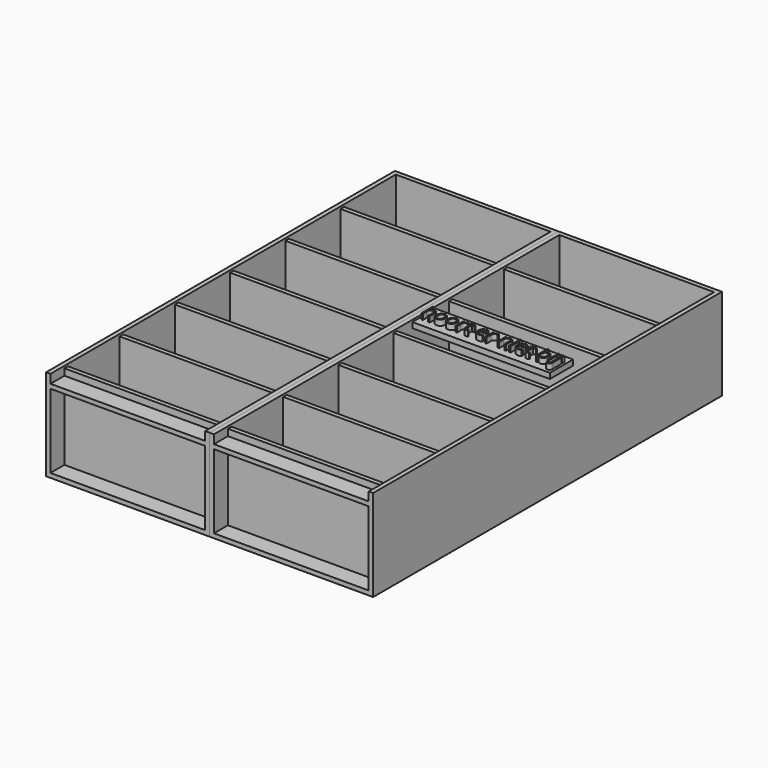
from build123d import *

# Parameters (mm, degrees)
F1_DEPTH      = 400
F3_W          = 630.7227015495
F3_H          = 132.8808516264
F4_DEPTH      = 25
F0_W          = 710
F0_H          = 20
F5_DEPTH      = 390
F6_W          = 710
F6_H          = 20
F7_DEPTH      = 80
F9_DEPTH      = 2000
F11_TEXT_SIZE = 85.9931443582
F12_DEPTH     = 25


# Not quite as in the source:
# - Text() gives the source's letters only with a copy of the font that has no kerning and outlines rounded to 1/6400 em; it was checked with that copy


with BuildPart() as f1:
    # F0 (on Top) → F1 (new body)
    with BuildSketch(Plane.XY):
        Polygon((355, -910), (355, -990), (375, -990), (375, 1010), (-375, 1010), (-375, -990), (-355, -990), (-355, -910), (-355, -890), (-355, -593.3333333333), (-355, -573.3333333333), (-355, -276.6666666667), (-355, -256.6666666667), (-355, 40), (-355, 60), (-355, 356.6666666667), (-355, 376.6666666667), (-355, 673.3333333333), (-355, 693.3333333333), (-355, 990), (355, 990), (355, 693.3333333333), (355, 673.3333333333), (355, 376.6666666667), (355, 356.6666666667), (355, 60), (355, 40), (355, -256.6666666667), (355, -276.6666666667), (355, -573.3333333333), (355, -593.3333333333), (355, -890), align=None)
    extrude(amount=F1_DEPTH)

    # F0 (on Top) → F5 (join, through all)
    with BuildSketch(Plane.XY):
        with Locations((0, 683.3333333333)):
            Rectangle(F0_W, F0_H)
        with Locations((0, 366.6666666667)):
            Rectangle(F0_W, F0_H)
        with Locations((0, 50)):
            Rectangle(F0_W, F0_H)
        with Locations((0, -266.6666666667)):
            Rectangle(F0_W, F0_H)
        with Locations((0, -583.3333333333)):
            Rectangle(F0_W, F0_H)
        with Locations((0, -900)):
            Rectangle(F0_W, F0_H)
    extrude(amount=F5_DEPTH)

    # F6 (on face) → F7 (join, through all)
    with BuildSketch(Plane.XZ.offset(990)):
        with Locations((0, 350)):
            Rectangle(F6_W, F6_H)
    extrude(amount=-F7_DEPTH)

    # F8 (on face) → F9 (join, through all)
    with BuildSketch(Plane.XZ.offset(990)):
        Polygon((375, -20), (375, 0), (355, 0), (-355, 0), (-375, 0), (-375, -20), align=None)
    extrude(amount=-F9_DEPTH)


with BuildPart() as f4:
    # F3 (on offset) → F4 (new body)
    with BuildSketch(Plane.XY.offset(390)):
        with Locations((-10.5079710484, 177.692271769)):
            Rectangle(F3_W, F3_H)
    extrude(amount=F4_DEPTH)

    # F11 (on face) → F12 (join)
    with BuildSketch(Plane.XY.offset(415)):
        with Locations((-320.8693218231, 146.7347398001)):
            Text('hoort er niet bij', F11_TEXT_SIZE, font='Open Sans', text_align=(TextAlign.LEFT, TextAlign.BOTTOM))
    extrude(amount=F12_DEPTH)


with BuildPart() as f10_1:
    # F10: instance of F1
    add(f1.part.mirror(Plane(origin=(-375, 10, 190), x_dir=(0, -1, 0), z_dir=(-1, 0, 0))))


solid = Compound([f1.part, f4.part, f10_1.part])
